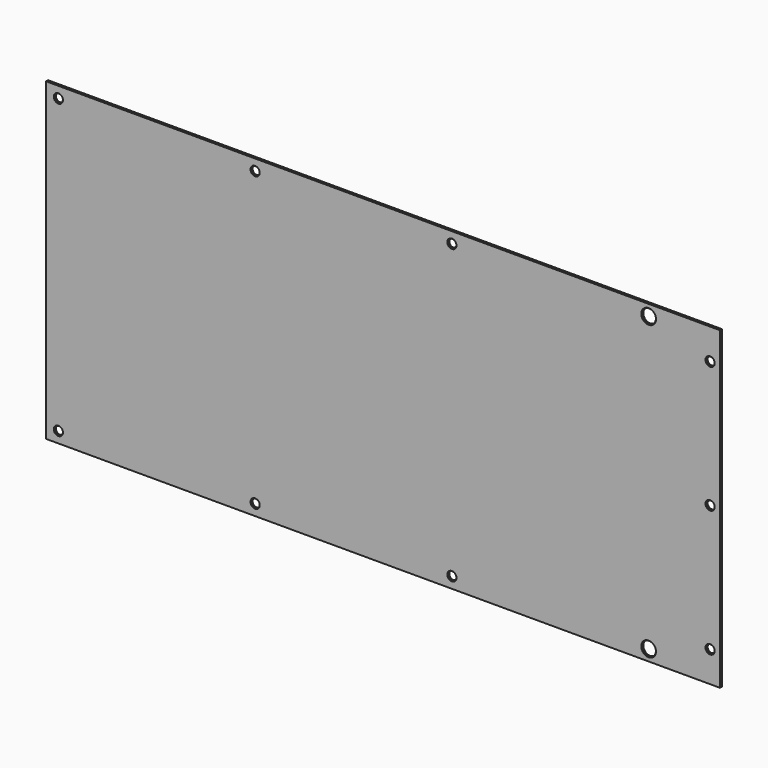
from build123d import *

# Parameters (mm, degrees)
F0_W     = 548
F0_H     = 256
F0_R     = 3.25
F0_R_2   = 5.5
F1_DEPTH = 2
F2_SIZE  = 0.5


with BuildPart() as f1:
    # F0 (on Front) → F1 (new body)
    with BuildSketch(Plane.XZ):
        Rectangle(F0_W, F0_H)
        with Locations((-264, -119)):
            Circle(F0_R, mode=Mode.SUBTRACT)
        with Locations((-104, -119)):
            Circle(F0_R, mode=Mode.SUBTRACT)
        with Locations((56, -119)):
            Circle(F0_R, mode=Mode.SUBTRACT)
        with Locations((216, -119)):
            Circle(F0_R_2, mode=Mode.SUBTRACT)
        with Locations((266, -103)):
            Circle(F0_R, mode=Mode.SUBTRACT)
        with Locations((-264, 119)):
            Circle(F0_R, mode=Mode.SUBTRACT)
        with Locations((-104, 119)):
            Circle(F0_R, mode=Mode.SUBTRACT)
        with Locations((266, 0)):
            Circle(F0_R, mode=Mode.SUBTRACT)
        with Locations((56, 119)):
            Circle(F0_R, mode=Mode.SUBTRACT)
        with Locations((266, 103)):
            Circle(F0_R, mode=Mode.SUBTRACT)
        with Locations((216, 119)):
            Circle(F0_R_2, mode=Mode.SUBTRACT)
    extrude(amount=F1_DEPTH)

    # F2
    f2_edges = [f1.edges().sort_by_distance(p)[0] for p in [
        (-260.75, -1, 119),
        (-267.25, 0, 119),
        (-267.25, -2, 119),
        (-100.75, -1, 119),
        (-107.25, 0, 119),
        (-107.25, -2, 119),
        (59.25, -1, 119),
        (52.75, 0, 119),
        (52.75, -2, 119),
        (269.25, -1, 103),
        (262.75, 0, 103),
        (262.75, -2, 103),
        (269.25, -1, 0),
        (262.75, 0, 0),
        (262.75, -2, 0),
        (269.25, -1, -103),
        (262.75, 0, -103),
        (262.75, -2, -103),
        (59.25, -1, -119),
        (52.75, 0, -119),
        (52.75, -2, -119),
        (-100.75, -1, -119),
        (-107.25, 0, -119),
        (-107.25, -2, -119),
        (-260.75, -1, -119),
        (-267.25, 0, -119),
        (-267.25, -2, -119),
        (221.5, -1, 119),
        (210.5, 0, 119),
        (210.5, -2, 119),
        (221.5, -1, -119),
        (210.5, 0, -119),
        (210.5, -2, -119),
    ]]
    chamfer(f2_edges, length=F2_SIZE)


solid = f1.part
